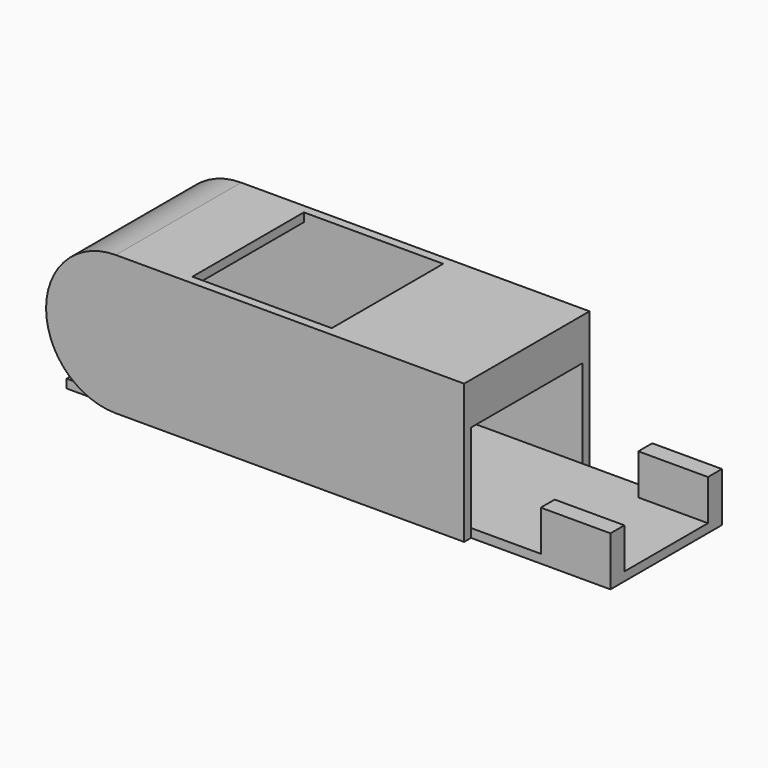
from build123d import *

# Parameters (mm, degrees)
F1_DEPTH = 19.05
F2_W     = 304.8
F2_H     = 92.075
F3_DEPTH = 304.8
F4_W     = 304.8
F4_H     = 92.075
F5_DEPTH = 19.05
F6_W     = 304.8
F6_H     = 19.05
F7_DEPTH = 304.8
F8_W     = 152.4
F8_H     = 38.1
F9_DEPTH = 88.9


# Not quite as in the source:
# - a feature names something its author has since deleted; it is built from what else it names


with BuildPart() as f1:
    # F0 (on Front) → F1 (new body)
    with BuildSketch(Plane.XZ):
        with BuildLine():
            Line((457.2, -152.4), (457.2, 152.4))
            Line((457.2, 152.4), (-304.8, 152.4))
            ThreePointArc((-304.8, 152.4), (-197.0369265472, 107.7630734528), (-152.4, 0))
            ThreePointArc((-152.4, 0), (-197.0369262947, -107.7630732004), (-304.799999286, -152.4))
            Line((-304.799999286, -152.4), (457.2, -152.4))
        make_face()
        with BuildLine():
            ThreePointArc((-152.4, 0), (-197.0369265472, 107.7630734528), (-304.8, 152.4))
            ThreePointArc((-304.8, 152.4), (-412.5630734984, 107.7630734073), (-457.2, -1.288e-07))
            ThreePointArc((-457.2, -1.288e-07), (-412.5630731549, -107.7630737508), (-304.799999286, -152.4))
            ThreePointArc((-304.799999286, -152.4), (-197.0369262947, -107.7630732004), (-152.4, 0))
        make_face()
    extrude(amount=F1_DEPTH)

    # F2 (on face) → F3 (join)
    with BuildSketch(Plane.XZ.offset(19.05)):
        with Locations((304.8, 106.3625)):
            Rectangle(F2_W, F2_H)
    extrude(amount=F3_DEPTH)

    # F4 (on face) → F5 (join)
    with BuildSketch(Plane.XZ.offset(323.85)):
        with BuildLine():
            Line((152.4, 60.325), (152.4, 152.4))
            Line((152.4, 152.4), (-304.8, 152.4))
            ThreePointArc((-304.8, 152.4), (-197.0369265472, 107.7630734528), (-152.4, 0))
            ThreePointArc((-152.4, 0), (-197.0369262947, -107.7630732004), (-304.799999286, -152.4))
            Line((-304.799999286, -152.4), (457.2, -152.4))
            Line((457.2, -152.4), (457.2, 60.325))
            Line((457.2, 60.325), (152.4, 60.325))
        make_face()
        with Locations((304.8, 106.3625)):
            Rectangle(F4_W, F4_H)
        with BuildLine():
            ThreePointArc((-152.4, 0), (-197.0369265472, 107.7630734528), (-304.8, 152.4))
            ThreePointArc((-304.8, 152.4), (-412.5630734984, 107.7630734073), (-457.2, -1.288e-07))
            ThreePointArc((-457.2, -1.288e-07), (-412.5630731549, -107.7630737508), (-304.799999286, -152.4))
            ThreePointArc((-304.799999286, -152.4), (-197.0369262947, -107.7630732004), (-152.4, 0))
        make_face()
    extrude(amount=F5_DEPTH)

    # F6 (on face) → F7 (join, through all)
    with BuildSketch(Plane.XZ.offset(19.05)):
        with BuildLine():
            ThreePointArc((-304.799999286, -152.4), (-342.8999996543, -147.5606655798), (-378.5803327453, -133.35))
            Line((-378.5803327453, -133.35), (-427.4579864061, -133.35))
            Line((-427.4579864061, -133.35), (-427.4579864061, -152.4))
            Line((-427.4579864061, -152.4), (-304.799999286, -152.4))
        make_face()
        with BuildLine():
            Line((-152.4, 133.35), (-152.4, 152.4))
            Line((-152.4, 152.4), (-304.8, 152.4))
            ThreePointArc((-304.8, 152.4), (-266.7, 147.5606654905), (-231.0196672547, 133.35))
            Line((-231.0196672547, 133.35), (-152.4, 133.35))
        make_face()
        with BuildLine():
            ThreePointArc((-231.0196672547, 133.35), (-266.7, 147.5606654905), (-304.8, 152.4))
            Line((-304.8, 152.4), (-304.8, 133.35))
            Line((-304.8, 133.35), (-231.0196672547, 133.35))
        make_face()
        with BuildLine():
            Line((-304.8, 133.35), (-304.8, 152.4))
            ThreePointArc((-304.8, 152.4), (-452.3606654905, 38.1), (-378.5803327453, -133.35))
            Line((-378.5803327453, -133.35), (-304.7999985066, -133.35))
            ThreePointArc((-304.7999985066, -133.35), (-438.15, -7.467e-07), (-304.8, 133.35))
        make_face()
        with BuildLine():
            Line((-304.7999985066, -133.35), (-378.5803327453, -133.35))
            ThreePointArc((-378.5803327453, -133.35), (-342.8999996543, -147.5606655798), (-304.799999286, -152.4))
            ThreePointArc((-304.799999286, -152.4), (-266.6999996543, -147.5606654012), (-231.0196672547, -133.35))
            Line((-231.0196672547, -133.35), (-304.7999985066, -133.35))
        make_face()
        with Locations((609.6, -142.875)):
            Rectangle(F6_W, F6_H)
        with BuildLine():
            ThreePointArc((-231.0196672547, -133.35), (-266.6999996543, -147.5606654012), (-304.799999286, -152.4))
            Line((-304.799999286, -152.4), (457.2, -152.4))
            Line((457.2, -152.4), (457.2, -133.35))
            Line((457.2, -133.35), (-231.0196672547, -133.35))
        make_face()
    extrude(amount=F7_DEPTH)

    # F8 (on face) → F9 (join)
    with BuildSketch(Plane.XY.offset(-133.35)):
        with Locations((685.8, -38.1)):
            Rectangle(F8_W, F8_H)
        with Locations((685.8, -304.8)):
            Rectangle(F8_W, F8_H)
    extrude(amount=F9_DEPTH)


solid = f1.part
